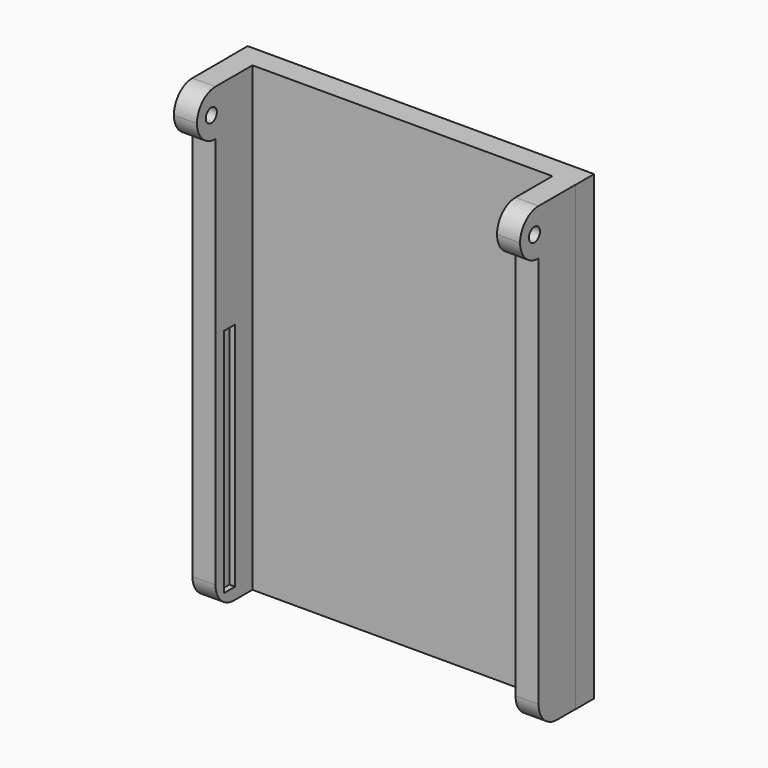
from build123d import *

# Parameters (mm, degrees)
F0_W     = 1500
F0_H     = 2000
F1_DEPTH = 100
F3_DEPTH = 100
F4_W     = 60
F4_H     = 1000
F5_DEPTH = 25
F7_R     = 30
F8_DEPTH = 1500.001
F9_R     = 99.99999


# Not quite as in the source:
# - a fillet or chamfer is up to 0.001 mm smaller than in the source, because OpenCascade refuses the exact size


with BuildPart() as f1:
    # F0 (on Front) → F1 (new body)
    with BuildSketch(Plane.XZ):
        with Locations((0.2205967903, 375.376350426)):
            Rectangle(F0_W, F0_H)
    extrude(amount=F1_DEPTH)

    # F2 (on face) → F3 (join)
    with BuildSketch(Plane(origin=(-749.7794032097, 0, 0), x_dir=(0, -1, 0), z_dir=(-1, 0, 0))):
        Polygon((400, 1375.376350426), (100, 1375.376350426), (100, -624.623649574), (300, -624.623649574), (300, 1175.376350426), (400, 1175.376350426), align=None)
    extrude(amount=-F3_DEPTH)

    # F4 (on face) → F5 (cut)
    with BuildSketch(Plane.YZ.offset(-649.7794032097)):
        with Locations((-223.8319441676, -74.623649574)):
            Rectangle(F4_W, F4_H)
    extrude(amount=-F5_DEPTH, mode=Mode.SUBTRACT)

    # F6: F1 across plane


with BuildPart() as f1_1:
    add(f1.part)
    add(f1.part.mirror(Plane.YZ))

    # F7 (on face) → F8 (cut, through all)
    with BuildSketch(Plane(origin=(-749.7794032097, 0, 0), x_dir=(0, -1, 0), z_dir=(-1, 0, 0))):
        with Locations((322.3870694637, 1275.376350426)):
            Circle(F7_R)
    extrude(amount=-F8_DEPTH, mode=Mode.SUBTRACT)

    # F9 (radius 100 in the source; OpenCascade refuses exactly that, so slightly less here)
    f9_edges = [f1_1.edges().sort_by_distance(p)[0] for p in [
        (-699.779403, -400, 1175.37635),
        (699.779403, -400, 1175.37635),
        (-699.779403, -300, -624.62365),
        (699.779403, -300, -624.62365),
        (699.779403, -400, 1375.37635),
        (-699.779403, -400, 1375.37635),
    ]]
    fillet(f9_edges, radius=F9_R)


solid = f1_1.part
